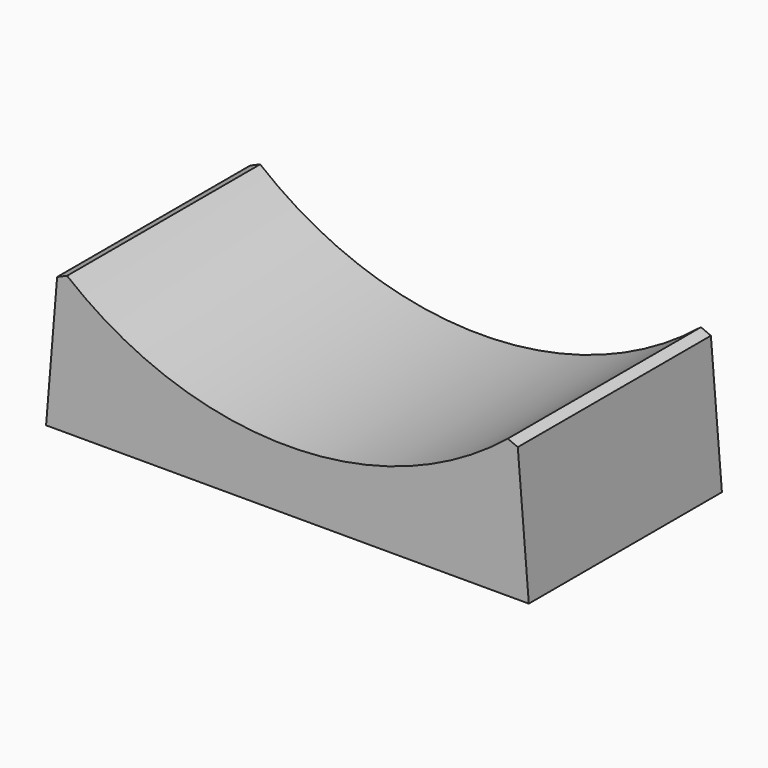
from build123d import *

# Parameters (mm, degrees)
F1_DEPTH    = 25.4
F2_T1_DEPTH = 31.742344746


# Not quite as in the source:
# - a fillet or chamfer that OpenCascade refuses, or shapes differently, is made with other operations: its cross-section is extruded or revolved along the edge and cut away or added


with BuildPart() as f1:
    # F0 (on Front) → F1 (new body)
    with BuildSketch(Plane.XZ):
        with BuildLine():
            Line((1.2633143634, 15.3614934534), (0, 0))
            Line((0, 0), (50.8, 0))
            Line((50.8, 0), (49.5366856366, 15.3614934534))
            ThreePointArc((49.5366856366, 15.3614934534), (25.4, 6.35), (1.2633143634, 15.3614934534))
        make_face()
    extrude(amount=F1_DEPTH)

    # F2: chamfer of 1.27 on 2 edges, made by hand

    # F2_s2 → F2_t1 (cut)
    with BuildSketch(Plane.XZ.offset(-3.171172373)):
        with BuildLine():
            Line((2.2549090841, 14.5889641953), (1.1146425309, 14.1017672287))
            Line((1.1146425309, 14.1017672287), (1.089327991, 14.103849072))
            ThreePointArc((1.089327991, 14.103849072), (1.1860490936, 14.7318712483), (1.2379998236, 15.3635752967))
            Line((1.2379998236, 15.3635752967), (1.2799603535, 15.3806786304))
            ThreePointArc((1.2799603535, 15.3806786304), (1.7575594643, 14.9733769005), (2.2709034327, 14.6086959162))
            Line((2.2709034327, 14.6086959162), (2.2549090841, 14.5889641953))
        make_face()
        with BuildLine():
            Line((48.5450909159, 14.5889641953), (49.6853574691, 14.1017672287))
            Line((49.6853574691, 14.1017672287), (49.710672009, 14.103849072))
            ThreePointArc((49.710672009, 14.103849072), (49.6139509064, 14.7318712483), (49.5620001764, 15.3635752967))
            Line((49.5620001764, 15.3635752967), (49.5200396465, 15.3806786304))
            ThreePointArc((49.5200396465, 15.3806786304), (49.0424405357, 14.9733769005), (48.5290965673, 14.6086959162))
            Line((48.5290965673, 14.6086959162), (48.5450909159, 14.5889641953))
        make_face()
    extrude(amount=F2_T1_DEPTH, mode=Mode.SUBTRACT)


solid = f1.part
